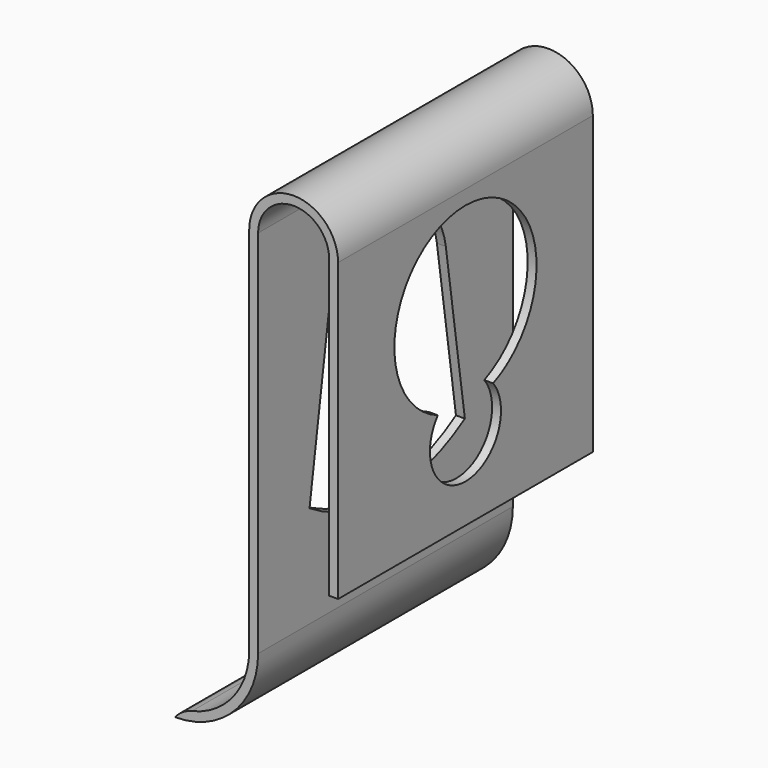
from build123d import *

# Parameters (mm, degrees)
F1_DEPTH    = 21.5
F3_DEPTH    = 1.80793
F5_DEPTH    = 2.4624
F6_T1_DEPTH = 27.2031140795


# Not quite as in the source:
# - a fillet or chamfer that OpenCascade refuses, or shapes differently, is made with other operations: its cross-section is extruded or revolved along the edge and cut away or added


with BuildPart() as f1:
    # F0 (on Front) → F1 (new body)
    with BuildSketch(Plane.XZ):
        with BuildLine():
            Line((0, 25), (0, 0))
            ThreePointArc((0, 0), (-1.4644660941, -3.5355339059), (-5, -5))
            Line((-5, -5), (-5, -5.6))
            ThreePointArc((-5, -5.6), (-1.0402020254, -3.9597979746), (0.6, 0))
            Line((0.6, 0), (0.6, 25))
            ThreePointArc((0.6, 25), (3, 27.4), (5.4, 25))
            Line((5.4, 25), (5.4, 5))
            Line((5.4, 5), (6, 5))
            Line((6, 5), (6, 25))
            ThreePointArc((6, 25), (3, 28), (0, 25))
        make_face()
    extrude(amount=F1_DEPTH)

    # F2 (on face) → F3 (cut)
    with BuildSketch(Plane(origin=(0, 0, 0), x_dir=(0, -1, 0), z_dir=(-1, 0, 0))):
        with BuildLine():
            Line((5.6591296673, 17.7571138706), (4.051160203, 6.875274219))
            ThreePointArc((4.051160203, 6.875274219), (10.605420418, 4.9272229372), (17.159680633, 6.875274219))
            Line((17.159680633, 6.875274219), (15.5517111687, 17.7571138706))
            ThreePointArc((15.5517111687, 17.7571138706), (10.605420418, 22.0262186595), (5.6591296673, 17.7571138706))
        make_face()
    extrude(amount=-F3_DEPTH, mode=Mode.SUBTRACT)

    # F4 (on face) → F5 (cut)
    with BuildSketch(Plane.YZ.offset(6)):
        with BuildLine():
            ThreePointArc((-13.0845142088, 12.5011450204), (-10.75, 7.6169891327), (-8.4154857912, 12.5011450204))
            ThreePointArc((-8.4154857912, 12.5011450204), (-10.75, 24.0283543894), (-13.0845142088, 12.5011450204))
        make_face()
    extrude(amount=-F5_DEPTH, mode=Mode.SUBTRACT)

    # F6: fillet of radius 2 on 1 edges, made by hand

    # F6_s2 → F6_t1 (cut)
    with BuildSketch(Plane.XZ.offset(-2.8515570398)):
        with BuildLine():
            ThreePointArc((-5, -5.6), (-4.4967757486, -5.136601148), (-3.8668213437, -4.8698979592))
            ThreePointArc((-3.8668213437, -4.8698979592), (-4.429688592, -4.9673680051), (-5, -5))
            Line((-5, -5), (-5, -5.6))
        make_face()
    extrude(amount=F6_T1_DEPTH, mode=Mode.SUBTRACT)


solid = f1.part
